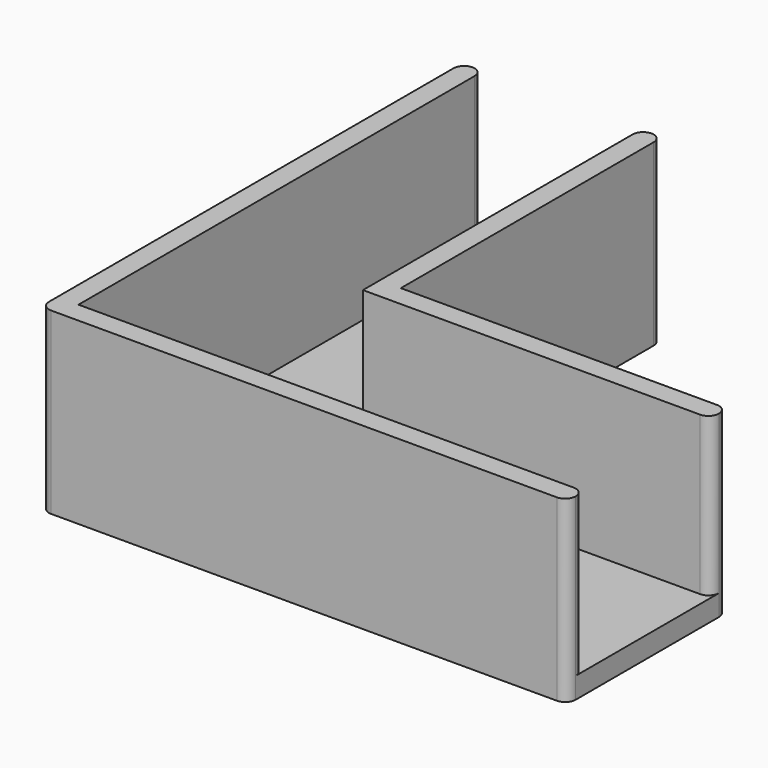
from build123d import *

# Parameters (mm, degrees)
F1_DEPTH = 17
F3_DEPTH = 15
F4_R     = 1.6
F5_DEPTH = 2
F6_R     = 0.99999
F8_DEPTH = 15
F9_R     = 3


# Not quite as in the source:
# - a fillet or chamfer is up to 0.001 mm smaller than in the source, because OpenCascade refuses the exact size


with BuildPart() as f1:
    # F0 (on Top) → F1 (new body)
    with BuildSketch(Plane.XY):
        Polygon((-6, 25), (-25, 25), (-25, -25), (25, -25), (25, -6), (9.5, -6), (-6, -6), (-6, 9.5), align=None)
        Polygon((9.5, -6), (-6, 9.5), (-6, -6), align=None)
    extrude(amount=F1_DEPTH)

    # F2 (on face) → F3 (cut)
    with BuildSketch(Plane.XY.offset(17)):
        Polygon((-8, 25), (-23, 25), (-23, -23), (25, -23), (25, -8), (-6, -8), (-8, -8), (-8, -6), align=None)
    extrude(amount=-F3_DEPTH, mode=Mode.SUBTRACT)

    # F4 (on face) → F5 (cut, through all)
    with BuildSketch(Plane(origin=(0, 0, 0), x_dir=(1, 0, 0), z_dir=(0, 0, -1))):
        with Locations((15, 15.5)):
            Circle(F4_R)
        with Locations((-5.5, 15.5)):
            Circle(F4_R)
        with Locations((-15.5, 5.5)):
            Circle(F4_R)
        with Locations((-15.5, -15)):
            Circle(F4_R)
    extrude(amount=-F5_DEPTH, mode=Mode.SUBTRACT)

    # F6 (radius 1 in the source; OpenCascade refuses exactly that, so slightly less here)
    f6_edges = [f1.edges().sort_by_distance(p)[0] for p in [
        (25, -25, 8.5),
        (25, -23, 9.5),
        (25, -8, 9.5),
        (25, -6, 8.5),
        (-25, -25, 8.5),
        (-25, 25, 8.5),
        (-8, 25, 9.5),
        (-23, 25, 9.5),
        (-6, 25, 8.5),
    ]]
    fillet(f6_edges, radius=F6_R)

    # F7 (on face) → F8 (cut)
    with BuildSketch(Plane.XY.offset(17)):
        Polygon((-6, -6), (9.5, -6), (-6, 9.5), align=None)
    extrude(amount=-F8_DEPTH, mode=Mode.SUBTRACT)

    # F9
    f9_edges = [f1.edges().sort_by_distance(p)[0] for p in [
        (-6, 9.5, 1),
        (9.5, -6, 1),
    ]]
    fillet(f9_edges, radius=F9_R)


solid = f1.part
